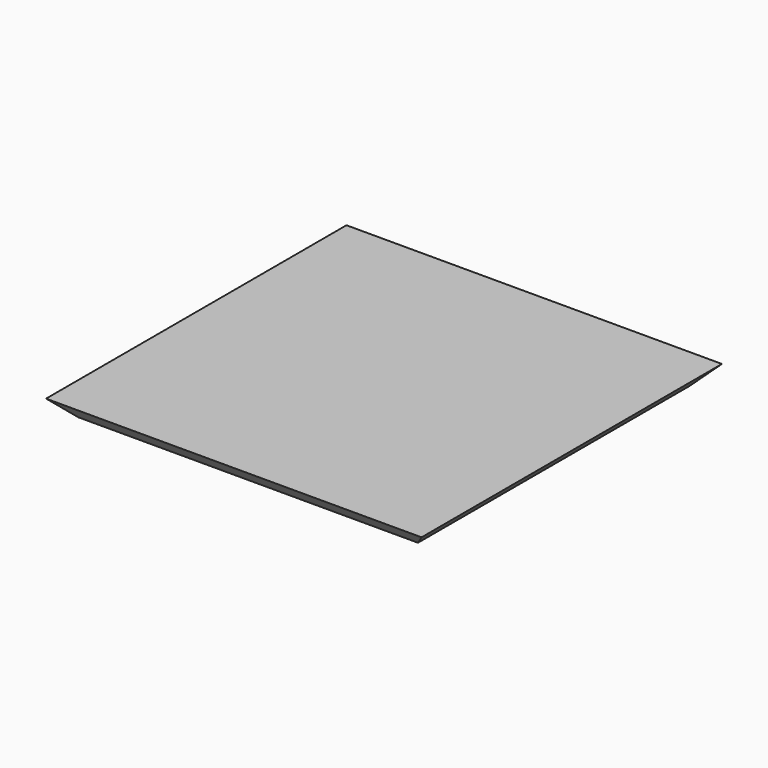
from build123d import *

# Parameters (mm, degrees)
F0_W     = 533.4
F0_H     = 533.4
F1_DEPTH = 25.4
F2_SIZE  = 25.39999


# Not quite as in the source:
# - a fillet or chamfer is up to 0.001 mm smaller than in the source, because OpenCascade refuses the exact size


with BuildPart() as f1:
    # F0 (on Top) → F1 (new body)
    with BuildSketch(Plane.XY):
        Rectangle(F0_W, F0_H)
    extrude(amount=F1_DEPTH)

    # F2 (size 25.4 in the source; OpenCascade refuses exactly that, so slightly less here)
    f2_edges = [f1.edges().sort_by_distance(p)[0] for p in [
        (266.7, 0, 0),
        (0, 266.7, 0),
        (-266.7, 0, 0),
        (0, -266.7, 0),
    ]]
    chamfer(f2_edges, length=F2_SIZE)


solid = f1.part
